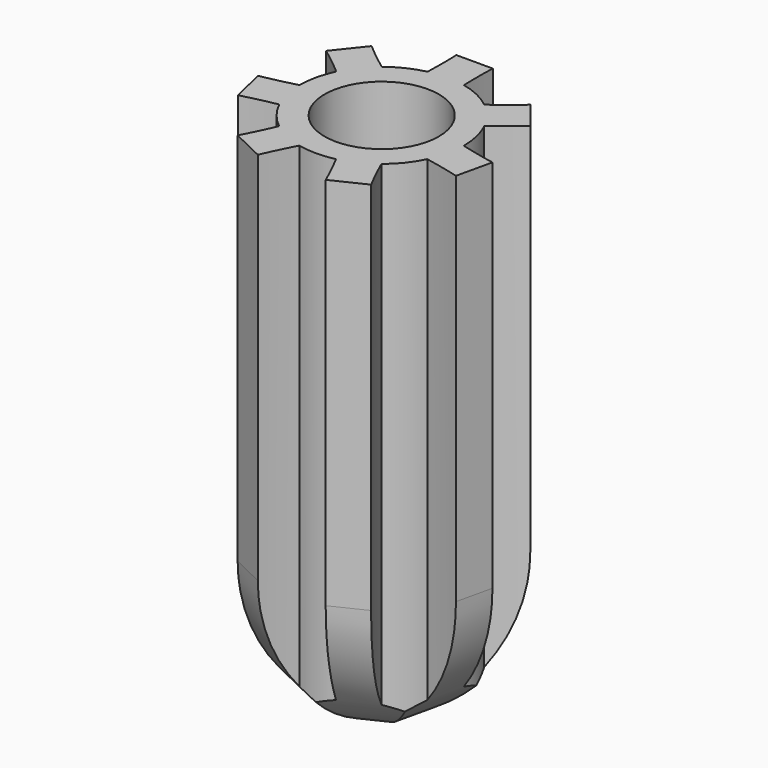
from build123d import *

# Parameters (mm, degrees)
F0_R         = 1.6
F1_DEPTH     = 15
F2_DEPTH     = 2
F3_T1_DEPTH  = 23.52
F3_T3_DEPTH  = 23.52
F3_T5_DEPTH  = 23.52
F3_T7_DEPTH  = 23.52
F3_T9_DEPTH  = 23.52
F3_T11_DEPTH = 23.52
F3_T13_DEPTH = 23.52


# Not quite as in the source:
# - a fillet or chamfer that OpenCascade refuses, or shapes differently, is made with other operations: its cross-section is extruded or revolved along the edge and cut away or added


with BuildPart() as f1:
    # F0 (on Top) → F1 (new body)
    with BuildSketch(Plane.XY):
        with BuildLine():
            ThreePointArc((-2.858932117, 1.6276078), (-2.4589449365, 1.3214191477), (-2.071427552, 0.9995938658))
            ThreePointArc((-2.071427552, 0.9995938658), (-2.242334198, 0.5117981481), (-2.2999992606, -0.0018442221))
            ThreePointArc((-2.2999992606, -0.0018442221), (-2.7887751164, -0.1236612902), (-3.2820013909, -0.2259798001))
            Line((-3.2820013909, -0.2259798001), (-3.0550300383, -1.2204062706))
            ThreePointArc((-3.0550300383, -1.2204062706), (-2.5662541825, -1.0985892024), (-2.073027908, -0.9962706925))
            ThreePointArc((-2.073027908, -0.9962706925), (-1.7982124097, -1.4340265443), (-1.4325842124, -1.7993616853))
            ThreePointArc((-1.4325842124, -1.7993616853), (-1.6420905549, -2.2574537369), (-1.8696162748, -2.7068681137))
            Line((-1.8696162748, -2.7068681137), (-0.9506280295, -3.1494295276))
            ThreePointArc((-0.9506280295, -3.1494295276), (-0.741121687, -2.691337476), (-0.5135959671, -2.2419230992))
            ThreePointArc((-0.5135959671, -2.2419230992), (0, -2.3), (0.5135959671, -2.2419230992))
            ThreePointArc((0.5135959671, -2.2419230992), (0.9979326, -2.0722283962), (1.4325842124, -1.7993616853))
            ThreePointArc((1.4325842124, -1.7993616853), (1.7982124097, -1.4340265443), (2.073027908, -0.9962706925))
            ThreePointArc((2.073027908, -0.9962706925), (2.242334198, -0.5117981481), (2.2999992606, -0.0018442221))
            ThreePointArc((2.2999992606, -0.0018442221), (2.242334198, 0.5117981481), (2.071427552, 0.9995938658))
            ThreePointArc((2.071427552, 0.9995938658), (2.4589449365, 1.3214191477), (2.858932117, 1.6276078))
            Line((2.858932117, 1.6276078), (2.2229725191, 2.4250759121))
            ThreePointArc((2.2229725191, 2.4250759121), (1.8354551346, 2.1032506302), (1.4354679542, 1.797061978))
            ThreePointArc((1.4354679542, 1.797061978), (0.9979326, 2.0722283962), (0.51, 2.2427438552))
            ThreePointArc((0.51, 2.2427438552), (0.5, 2.7463719276), (0.51, 3.25))
            Line((0.51, 3.25), (-0.51, 3.25))
            ThreePointArc((-0.51, 3.25), (-0.5, 2.7463719276), (-0.51, 2.2427438552))
            ThreePointArc((-0.51, 2.2427438552), (-0.9979326, 2.0722283962), (-1.4354679542, 1.797061978))
            ThreePointArc((-1.4354679542, 1.797061978), (-1.8354551346, 2.1032506302), (-2.2229725191, 2.4250759121))
            Line((-2.2229725191, 2.4250759121), (-2.858932117, 1.6276078))
        make_face()
        Circle(F0_R, mode=Mode.SUBTRACT)
        with BuildLine():
            ThreePointArc((2.2999992606, -0.0018442221), (2.242334198, -0.5117981481), (2.073027908, -0.9962706925))
            ThreePointArc((2.073027908, -0.9962706925), (2.5662541825, -1.0985892024), (3.0550300383, -1.2204062706))
            Line((3.0550300383, -1.2204062706), (3.2820013909, -0.2259798001))
            ThreePointArc((3.2820013909, -0.2259798001), (2.7887751164, -0.1236612902), (2.2999992606, -0.0018442221))
        make_face()
        with BuildLine():
            ThreePointArc((1.4325842124, -1.7993616853), (0.9979326, -2.0722283962), (0.5135959671, -2.2419230992))
            ThreePointArc((0.5135959671, -2.2419230992), (0.741121687, -2.691337476), (0.9506280295, -3.1494295276))
            Line((0.9506280295, -3.1494295276), (1.8696162748, -2.7068681137))
            ThreePointArc((1.8696162748, -2.7068681137), (1.6420905549, -2.2574537369), (1.4325842124, -1.7993616853))
        make_face()
    extrude(amount=F1_DEPTH)

    # F0 (on Top) → F2 (join)
    with BuildSketch(Plane.XY):
        Circle(F0_R)
    extrude(amount=F2_DEPTH)

    # F3: fillet of radius 4.5 on 7 edges, made by hand

    # F3_s2 → F3_t1 (cut)
    with BuildSketch(Plane(origin=(-10.5953938865, -5.102472772, 0), x_dir=(0, 0, 1), z_dir=(0.9009688679, 0.4338837391, 0))):
        with BuildLine():
            ThreePointArc((0, -1.25), (1.3180194847, 1.9319805153), (4.5, 3.25))
            Line((4.5, 3.25), (0, 3.25))
            Line((0, 3.25), (0, -1.25))
        make_face()
    extrude(amount=F3_T1_DEPTH, mode=Mode.SUBTRACT)

    # F3_s4 → F3_t3 (cut)
    with BuildSketch(Plane(origin=(-10.5953938865, 5.102472772, 0), x_dir=(0, 0, 1), z_dir=(0.9009688679, -0.4338837391, 0))):
        with BuildLine():
            ThreePointArc((0, -1.25), (1.3180194847, 1.9319805153), (4.5, 3.25))
            Line((4.5, 3.25), (0, 3.25))
            Line((0, 3.25), (0, -1.25))
        make_face()
    extrude(amount=F3_T3_DEPTH, mode=Mode.SUBTRACT)

    # F3_s6 → F3_t5 (cut)
    with BuildSketch(Plane(origin=(-2.6168461833, 11.4651522473, 0), x_dir=(0, 0, 1), z_dir=(0.222520934, -0.9749279122, 0))):
        with BuildLine():
            ThreePointArc((0, -1.25), (1.3180194847, 1.9319805153), (4.5, 3.25))
            Line((4.5, 3.25), (0, 3.25))
            Line((0, 3.25), (0, -1.25))
        make_face()
    extrude(amount=F3_T5_DEPTH, mode=Mode.SUBTRACT)

    # F3_s8 → F3_t7 (cut)
    with BuildSketch(Plane(origin=(7.3322400699, 9.1943382338, 0), x_dir=(0, 0, 1), z_dir=(-0.6234898019, -0.7818314825, 0))):
        with BuildLine():
            ThreePointArc((4.5, 3.25), (1.3180194847, 1.9319805153), (0, -1.25))
            Line((0, -1.25), (0, 3.25))
            Line((0, 3.25), (4.5, 3.25))
        make_face()
    extrude(amount=F3_T7_DEPTH, mode=Mode.SUBTRACT)

    # F3_s10 → F3_t9 (cut)
    with BuildSketch(Plane.YZ.offset(-11.76)):
        with BuildLine():
            ThreePointArc((-1.25, 0), (1.9319805153, 1.3180194847), (3.25, 4.5))
            Line((3.25, 4.5), (3.25, 0))
            Line((3.25, 0), (-1.25, 0))
        make_face()
    extrude(amount=F3_T9_DEPTH, mode=Mode.SUBTRACT)

    # F3_s12 → F3_t11 (cut)
    with BuildSketch(Plane(origin=(7.3322400699, -9.1943382338, 0), x_dir=(0, 0, 1), z_dir=(-0.6234898019, 0.7818314825, 0))):
        with BuildLine():
            ThreePointArc((0, -1.25), (1.3180194847, 1.9319805153), (4.5, 3.25))
            Line((4.5, 3.25), (0, 3.25))
            Line((0, 3.25), (0, -1.25))
        make_face()
    extrude(amount=F3_T11_DEPTH, mode=Mode.SUBTRACT)

    # F3_s14 → F3_t13 (cut)
    with BuildSketch(Plane(origin=(-2.6168461833, -11.4651522473, 0), x_dir=(0, 0, 1), z_dir=(0.222520934, 0.9749279122, 0))):
        with BuildLine():
            ThreePointArc((0, -1.25), (1.3180194847, 1.9319805153), (4.5, 3.25))
            Line((4.5, 3.25), (0, 3.25))
            Line((0, 3.25), (0, -1.25))
        make_face()
    extrude(amount=F3_T13_DEPTH, mode=Mode.SUBTRACT)


solid = f1.part
